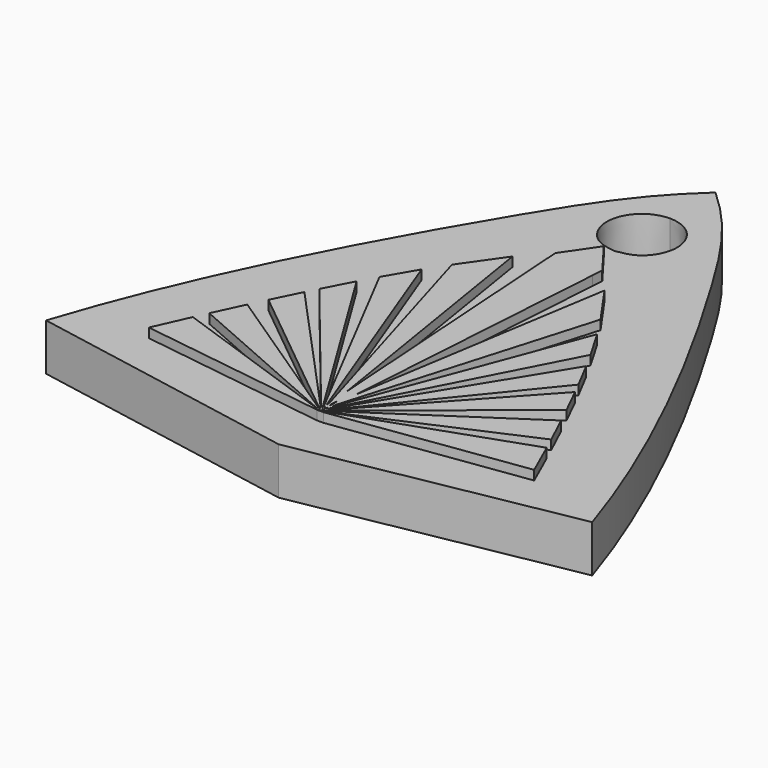
from build123d import *

# Parameters (mm, degrees)
F1_DEPTH = 5
F2_DEPTH = 6


# Not quite as in the source:
# - ends of sketch curves that miss each other by under 0.0002 mm in the source are joined
# - the dataset's text gives a spline's control points without its knots; the knots are read off the source's solid


with BuildPart() as f1:
    # F0 (on Top) → F1 (new body)
    with BuildSketch(Plane.XY):
        with BuildLine():
            add(Edge.make_bspline(
                [(0, 28.767477721), (-4.3973337825, 24.7953766473), (-10.7954077038, 15.1380571302), (-24.0578016888, -8.5453422723), (-29.069265, -23.969107)],
                knots=[0, 0, 0, 0, 0.3845016871, 1, 1, 1, 1], degree=3))
            Line((-29.069265, -23.969107), (-0.0365, -29.314396))
            Line((-0.0365, -29.314396), (29.069265, -23.969107))
            add(Edge.make_bspline(
                [(0, 28.767477721), (4.3973337825, 24.7953766473), (10.7954077038, 15.1380571302), (24.0578016888, -8.5453422723), (29.069265, -23.969107)],
                knots=[0, 0, 0, 0, 0.3845016871, 1, 1, 1, 1], degree=3))
        make_face()
        with BuildLine():
            Line((0.319138, -23.880866), (0.319138, -23.884253))
            Line((0.319138, -23.884253), (18.947309, -17.376961))
            add(Edge.make_bspline(
                [(20.618817, -21.132774), (20.455632, -20.760303), (20.108363, -19.967658), (19.551311, -18.715647), (19.15498, -17.837234), (18.947309, -17.376961)],
                knots=[0, 0, 0, 0, 1.219947, 2.596139, 4.110998, 4.110998, 4.110998, 4.110998], degree=3))
            Line((20.618817, -21.132774), (0.447831, -23.968919))
            Line((0.447831, -23.968919), (0.312364, -23.968919))
            Line((0.312364, -23.968919), (0.280003, -23.968919))
            Line((0.280003, -23.968919), (0.275111, -23.968919))
            Line((0.275111, -23.968919), (0.254791, -23.968919))
            Line((0.254791, -23.968919), (0.244631, -23.968919))
            Line((0.244631, -23.968919), (-0.019905, -23.968919))
            Line((-0.019905, -23.968919), (-0.030065, -23.968919))
            Line((-0.030065, -23.968919), (-0.04888, -23.968919))
            Line((-0.04888, -23.968919), (-0.054148, -23.968919))
            Line((-0.054148, -23.968919), (-0.086134, -23.968919))
            Line((-0.086134, -23.968919), (-0.2216, -23.968919))
            Line((-0.2216, -23.968919), (-20.392586, -21.132774))
            add(Edge.make_bspline(
                [(-18.721078, -17.376961), (-18.928749, -17.837234), (-19.32508, -18.715647), (-19.882132, -19.967658), (-20.229401, -20.760303), (-20.392586, -21.132774)],
                knots=[0, 0, 0, 0, 1.514859, 2.891051, 4.110998, 4.110998, 4.110998, 4.110998], degree=3))
            Line((-18.721078, -17.376961), (-0.092907, -23.884253))
            Line((-0.092907, -23.884253), (-0.092907, -23.880866))
            Line((-0.092907, -23.880866), (-18.083632, -15.981654))
            add(Edge.make_bspline(
                [(-16.595004, -12.792543), (-16.767405, -13.156812), (-17.107374, -13.875134), (-17.603121, -14.938403), (-17.925311, -15.637919), (-18.083632, -15.981654)],
                knots=[0, 0, 0, 0, 1.209017, 2.384129, 3.51946, 3.51946, 3.51946, 3.51946], degree=3))
            Line((-16.595004, -12.792543), (-0.09968, -23.772493))
            Line((-0.09968, -23.772493), (-0.101185, -23.736744))
            Line((-0.101185, -23.736744), (-15.752101, -11.0311))
            add(Edge.make_bspline(
                [(-14.292447, -8.070777), (-14.458037, -8.401363), (-14.788026, -9.060156), (-15.273718, -10.047373), (-15.593176, -10.704294), (-15.752101, -11.0311)],
                knots=[0, 0, 0, 0, 1.109215, 2.210448, 3.300648, 3.300648, 3.300648, 3.300648], degree=3))
            Line((-14.292447, -8.070777), (-0.111722, -23.597891))
            Line((-0.111722, -23.597891), (-0.113227, -23.56553))
            Line((-0.113227, -23.56553), (-13.678708, -6.854964))
            add(Edge.make_bspline(
                [(-12.106918, -3.854377), (-12.283656, -4.184869), (-12.638061, -4.847592), (-13.161704, -5.84798), (-13.506245, -6.519052), (-13.678708, -6.854964)],
                knots=[0, 0, 0, 0, 1.124341, 2.254598, 3.387391, 3.387391, 3.387391, 3.387391], degree=3))
            Line((-12.106918, -3.854377), (-0.126774, -23.361953))
            Line((-0.126774, -23.361953), (-0.136934, -23.211058))
            Line((-0.136934, -23.211058), (-11.115001, -2.041758))
            add(Edge.make_bspline(
                [(-9.227876, 1.200034), (-9.438006, 0.852886), (-9.864261, 0.148687), (-10.492017, -0.932835), (-10.905719, -1.669232), (-11.115001, -2.041758)],
                knots=[0, 0, 0, 0, 1.217356, 2.469433, 3.75129, 3.75129, 3.75129, 3.75129], degree=3))
            Line((-9.227876, 1.200034), (-0.164027, -22.805787))
            Line((-0.164027, -22.805787), (-0.194507, -22.35649))
            Line((-0.194507, -22.35649), (-7.79381, 3.443136))
            add(Edge.make_bspline(
                [(-4.787579, 7.734419), (-5.135061, 7.252834), (-5.826681, 6.294297), (-6.832139, 4.866004), (-7.477648, 3.910923), (-7.79381, 3.443136)],
                knots=[0, 0, 0, 0, 1.781576, 3.546009, 5.239803, 5.239803, 5.239803, 5.239803], degree=3))
            Line((-4.787579, 7.734419), (-0.367603, -19.764184))
            Line((-0.367603, -19.764184), (-2.305529, 9.216274))
            Line((-2.305529, 9.216274), (-2.378154, 10.418917))
            Line((-2.378154, 10.418917), (-2.359716, 10.440366))
            Line((-2.359716, 10.440366), (-2.381541, 10.440366))
            Line((-2.381541, 10.440366), (-0.010122, 13.91772))
            Line((-0.010122, 13.91772), (2.610782, 10.440366))
            Line((2.610782, 10.440366), (2.585946, 10.440366))
            Line((2.585946, 10.440366), (2.604761, 10.418917))
            Line((2.604761, 10.418917), (2.53176, 9.216274))
            Line((2.53176, 9.216274), (0.593834, -19.764184))
            Line((0.593834, -19.764184), (5.011929, 7.734419))
            add(Edge.make_bspline(
                [(8.020041, 3.443136), (7.703893, 3.910928), (7.058366, 4.866089), (6.052566, 6.294592), (5.359965, 7.252875), (5.011929, 7.734419)],
                knots=[0, 0, 0, 0, 1.693786, 3.458451, 5.240898, 5.240898, 5.240898, 5.240898], degree=3))
            Line((8.020041, 3.443136), (0.420738, -22.35649))
            Line((0.420738, -22.35649), (0.390258, -22.805787))
            Line((0.390258, -22.805787), (9.454106, 1.200034))
            add(Edge.make_bspline(
                [(11.341608, -2.041758), (11.132228, -1.669238), (10.718345, -0.932874), (10.090504, 0.148671), (9.664238, 0.852884), (9.454106, 1.200034)],
                knots=[0, 0, 0, 0, 1.281987, 2.534113, 3.751476, 3.751476, 3.751476, 3.751476], degree=3))
            Line((11.341608, -2.041758), (0.363164, -23.211058))
            Line((0.363164, -23.211058), (0.353004, -23.361953))
            Line((0.353004, -23.361953), (12.333149, -3.854377))
            add(Edge.make_bspline(
                [(13.904939, -6.854964), (13.732109, -6.519097), (13.386923, -5.848287), (12.86394, -4.84756), (12.509769, -4.184858), (12.333149, -3.854377)],
                knots=[0, 0, 0, 0, 1.133177, 2.263239, 3.387384, 3.387384, 3.387384, 3.387384], degree=3))
            Line((13.904939, -6.854964), (0.339458, -23.56553))
            Line((0.339458, -23.56553), (0.337576, -23.597891))
            Line((0.337576, -23.597891), (14.518678, -8.070777))
            add(Edge.make_bspline(
                [(15.978331, -11.0311), (15.819406, -10.704294), (15.499948, -10.047374), (15.014257, -9.060156), (14.684268, -8.401363), (14.518678, -8.070777)],
                knots=[0, 0, 0, 0, 1.0902, 2.191433, 3.300648, 3.300648, 3.300648, 3.300648], degree=3))
            Line((15.978331, -11.0311), (0.327792, -23.736744))
            Line((0.327792, -23.736744), (0.325911, -23.772493))
            Line((0.325911, -23.772493), (16.821235, -12.792543))
            add(Edge.make_bspline(
                [(18.309863, -15.981654), (18.151542, -15.637919), (17.829352, -14.938403), (17.333605, -13.875134), (16.993636, -13.156812), (16.821235, -12.792543)],
                knots=[0, 0, 0, 0, 1.135331, 2.310443, 3.51946, 3.51946, 3.51946, 3.51946], degree=3))
            Line((18.309863, -15.981654), (0.319138, -23.880866))
        make_face(mode=Mode.SUBTRACT)
        with BuildLine():
            add(Edge.make_bspline(
                [(-0.036575, 15.295228), (0.621493, 15.39784), (1.918116, 15.600022), (3.345493, 17.086348), (3.874317, 19.025119), (3.345531, 20.984289), (1.918153, 22.410914), (0.6214109026, 22.762095581), (-0.0367424704, 22.7620752759), (-0.0368262533, 22.7620752704)],
                knots=[0, 0, 0, 0, 1.951831, 3.845791, 5.797691, 7.749847, 9.643876, 11.595711, 11.5959595, 11.5959595, 11.5959595, 11.5959595], degree=3))
            add(Edge.make_bspline(
                [(-0.0368262533, 22.7620752704), (-0.6948437512, 22.7620322819), (-1.9914531815, 22.4108298617), (-3.418944, 20.984346), (-3.947897, 19.025119), (-3.418906, 17.086291), (-1.991357, 15.60004), (-0.694669, 15.397845), (-0.036575, 15.295228)],
                knots=[11.5959595, 11.5959595, 11.5959595, 11.5959595, 13.54764, 15.441797, 17.393979, 19.345905, 21.239993, 23.191919, 23.191919, 23.191919, 23.191919], degree=3))
        make_face(mode=Mode.SUBTRACT)
    extrude(amount=F1_DEPTH)

    # F0 (on Top) → F2 (join)
    with BuildSketch(Plane.XY):
        with BuildLine():
            Line((18.947309, -17.376961), (0.319138, -23.884253))
            Line((0.319138, -23.884253), (0.319138, -23.880866))
            Line((0.319138, -23.880866), (18.309863, -15.981654))
            add(Edge.make_bspline(
                [(18.309863, -15.981654), (18.151542, -15.637919), (17.829352, -14.938403), (17.333605, -13.875134), (16.993636, -13.156812), (16.821235, -12.792543)],
                knots=[0, 0, 0, 0, 1.135331, 2.310443, 3.51946, 3.51946, 3.51946, 3.51946], degree=3))
            Line((16.821235, -12.792543), (0.325911, -23.772493))
            Line((0.325911, -23.772493), (0.327792, -23.736744))
            Line((0.327792, -23.736744), (15.978331, -11.0311))
            add(Edge.make_bspline(
                [(15.978331, -11.0311), (15.819406, -10.704294), (15.499948, -10.047374), (15.014257, -9.060156), (14.684268, -8.401363), (14.518678, -8.070777)],
                knots=[0, 0, 0, 0, 1.0902, 2.191433, 3.300648, 3.300648, 3.300648, 3.300648], degree=3))
            Line((14.518678, -8.070777), (0.337576, -23.597891))
            Line((0.337576, -23.597891), (0.339458, -23.56553))
            Line((0.339458, -23.56553), (13.904939, -6.854964))
            add(Edge.make_bspline(
                [(13.904939, -6.854964), (13.732109, -6.519097), (13.386923, -5.848287), (12.86394, -4.84756), (12.509769, -4.184858), (12.333149, -3.854377)],
                knots=[0, 0, 0, 0, 1.133177, 2.263239, 3.387384, 3.387384, 3.387384, 3.387384], degree=3))
            Line((12.333149, -3.854377), (0.353004, -23.361953))
            Line((0.353004, -23.361953), (0.363164, -23.211058))
            Line((0.363164, -23.211058), (11.341608, -2.041758))
            add(Edge.make_bspline(
                [(11.341608, -2.041758), (11.132228, -1.669238), (10.718345, -0.932874), (10.090504, 0.148671), (9.664238, 0.852884), (9.454106, 1.200034)],
                knots=[0, 0, 0, 0, 1.281987, 2.534113, 3.751476, 3.751476, 3.751476, 3.751476], degree=3))
            Line((9.454106, 1.200034), (0.390258, -22.805787))
            Line((0.390258, -22.805787), (0.420738, -22.35649))
            Line((0.420738, -22.35649), (8.020041, 3.443136))
            add(Edge.make_bspline(
                [(8.020041, 3.443136), (7.703893, 3.910928), (7.058366, 4.866089), (6.052566, 6.294592), (5.359965, 7.252875), (5.011929, 7.734419)],
                knots=[0, 0, 0, 0, 1.693786, 3.458451, 5.240898, 5.240898, 5.240898, 5.240898], degree=3))
            Line((5.011929, 7.734419), (0.593834, -19.764184))
            Line((0.593834, -19.764184), (2.53176, 9.216274))
            Line((2.53176, 9.216274), (2.604761, 10.418917))
            Line((2.604761, 10.418917), (2.585946, 10.440366))
            Line((2.585946, 10.440366), (2.610782, 10.440366))
            Line((2.610782, 10.440366), (-0.010122, 13.91772))
            Line((-0.010122, 13.91772), (-2.381541, 10.440366))
            Line((-2.381541, 10.440366), (-2.359716, 10.440366))
            Line((-2.359716, 10.440366), (-2.378154, 10.418917))
            Line((-2.378154, 10.418917), (-2.305529, 9.216274))
            Line((-2.305529, 9.216274), (-0.367603, -19.764184))
            Line((-0.367603, -19.764184), (-4.787579, 7.734419))
            add(Edge.make_bspline(
                [(-4.787579, 7.734419), (-5.135061, 7.252834), (-5.826681, 6.294297), (-6.832139, 4.866004), (-7.477648, 3.910923), (-7.79381, 3.443136)],
                knots=[0, 0, 0, 0, 1.781576, 3.546009, 5.239803, 5.239803, 5.239803, 5.239803], degree=3))
            Line((-7.79381, 3.443136), (-0.194507, -22.35649))
            Line((-0.194507, -22.35649), (-0.164027, -22.805787))
            Line((-0.164027, -22.805787), (-9.227876, 1.200034))
            add(Edge.make_bspline(
                [(-9.227876, 1.200034), (-9.438006, 0.852886), (-9.864261, 0.148687), (-10.492017, -0.932835), (-10.905719, -1.669232), (-11.115001, -2.041758)],
                knots=[0, 0, 0, 0, 1.217356, 2.469433, 3.75129, 3.75129, 3.75129, 3.75129], degree=3))
            Line((-11.115001, -2.041758), (-0.136934, -23.211058))
            Line((-0.136934, -23.211058), (-0.126774, -23.361953))
            Line((-0.126774, -23.361953), (-12.106918, -3.854377))
            add(Edge.make_bspline(
                [(-12.106918, -3.854377), (-12.283656, -4.184869), (-12.638061, -4.847592), (-13.161704, -5.84798), (-13.506245, -6.519052), (-13.678708, -6.854964)],
                knots=[0, 0, 0, 0, 1.124341, 2.254598, 3.387391, 3.387391, 3.387391, 3.387391], degree=3))
            Line((-13.678708, -6.854964), (-0.113227, -23.56553))
            Line((-0.113227, -23.56553), (-0.111722, -23.597891))
            Line((-0.111722, -23.597891), (-14.292447, -8.070777))
            add(Edge.make_bspline(
                [(-14.292447, -8.070777), (-14.458037, -8.401363), (-14.788026, -9.060156), (-15.273718, -10.047373), (-15.593176, -10.704294), (-15.752101, -11.0311)],
                knots=[0, 0, 0, 0, 1.109215, 2.210448, 3.300648, 3.300648, 3.300648, 3.300648], degree=3))
            Line((-15.752101, -11.0311), (-0.101185, -23.736744))
            Line((-0.101185, -23.736744), (-0.09968, -23.772493))
            Line((-0.09968, -23.772493), (-16.595004, -12.792543))
            add(Edge.make_bspline(
                [(-16.595004, -12.792543), (-16.767405, -13.156812), (-17.107374, -13.875134), (-17.603121, -14.938403), (-17.925311, -15.637919), (-18.083632, -15.981654)],
                knots=[0, 0, 0, 0, 1.209017, 2.384129, 3.51946, 3.51946, 3.51946, 3.51946], degree=3))
            Line((-18.083632, -15.981654), (-0.092907, -23.880866))
            Line((-0.092907, -23.880866), (-0.092907, -23.884253))
            Line((-0.092907, -23.884253), (-18.721078, -17.376961))
            add(Edge.make_bspline(
                [(-18.721078, -17.376961), (-18.928749, -17.837234), (-19.32508, -18.715647), (-19.882132, -19.967658), (-20.229401, -20.760303), (-20.392586, -21.132774)],
                knots=[0, 0, 0, 0, 1.514859, 2.891051, 4.110998, 4.110998, 4.110998, 4.110998], degree=3))
            Line((-20.392586, -21.132774), (-0.2216, -23.968919))
            Line((-0.2216, -23.968919), (-0.086134, -23.968919))
            Line((-0.086134, -23.968919), (-0.054148, -23.968919))
            Line((-0.054148, -23.968919), (-0.04888, -23.968919))
            Line((-0.04888, -23.968919), (-0.030065, -23.968919))
            Line((-0.030065, -23.968919), (-0.019905, -23.968919))
            Line((-0.019905, -23.968919), (0.244631, -23.968919))
            Line((0.244631, -23.968919), (0.254791, -23.968919))
            Line((0.254791, -23.968919), (0.275111, -23.968919))
            Line((0.275111, -23.968919), (0.280003, -23.968919))
            Line((0.280003, -23.968919), (0.312364, -23.968919))
            Line((0.312364, -23.968919), (0.447831, -23.968919))
            Line((0.447831, -23.968919), (20.618817, -21.132774))
            add(Edge.make_bspline(
                [(20.618817, -21.132774), (20.455632, -20.760303), (20.108363, -19.967658), (19.551311, -18.715647), (19.15498, -17.837234), (18.947309, -17.376961)],
                knots=[0, 0, 0, 0, 1.219947, 2.596139, 4.110998, 4.110998, 4.110998, 4.110998], degree=3))
        make_face()
        Polygon((0.000415, -23.840226), (-0.013132, -23.830066), (-0.00824, -23.813133), (0.005306, -23.824798), align=None, mode=Mode.SUBTRACT)
        Polygon((-0.015014, -23.546715), (-0.023292, -23.531663), (-0.016519, -23.445115), (-0.002972, -23.472208), align=None, mode=Mode.SUBTRACT)
        Polygon((0.112175, -23.914733), (0.110669, -23.913227), (0.112175, -23.911346), (0.115561, -23.913227), align=None, mode=Mode.SUBTRACT)
        Polygon((0.042936, -23.867319), (0.027508, -23.859041), (0.034281, -23.846999), (0.047828, -23.859041), align=None, mode=Mode.SUBTRACT)
        Polygon((0.080189, -23.806359), (0.06288, -23.789426), (0.064761, -23.786039), (0.081695, -23.804478), align=None, mode=Mode.SUBTRACT)
        Polygon((0.183671, -23.867319), (0.178403, -23.859041), (0.191949, -23.846999), (0.198723, -23.859041), align=None, mode=Mode.SUBTRACT)
        Polygon((0.146041, -23.806359), (0.144536, -23.804478), (0.159588, -23.786039), (0.161469, -23.789426), align=None, mode=Mode.SUBTRACT)
        Polygon((0.032776, -23.753678), (0.013961, -23.735239), (0.017348, -23.724703), (0.034281, -23.746904), align=None, mode=Mode.SUBTRACT)
        Polygon((0.112175, -23.753678), (0.097123, -23.726584), (0.112175, -23.694223), (0.129108, -23.726584), align=None, mode=Mode.SUBTRACT)
        Polygon((0.208883, -23.724703), (0.212269, -23.735239), (0.193455, -23.753678), (0.190444, -23.746904), align=None, mode=Mode.SUBTRACT)
        Polygon((0.225816, -23.840226), (0.220548, -23.824798), (0.234471, -23.813133), (0.239363, -23.830066), align=None, mode=Mode.SUBTRACT)
        Polygon((0.080189, -23.629876), (0.06288, -23.672774), (0.042936, -23.638531), (0.057988, -23.587731), align=None, mode=Mode.SUBTRACT)
        Polygon((0.183671, -23.638531), (0.162975, -23.672774), (0.146041, -23.629876), (0.168243, -23.587731), align=None, mode=Mode.SUBTRACT)
        Polygon((0.112175, -23.541823), (0.090349, -23.478981), (0.112175, -23.399207), (0.135881, -23.478981), align=None, mode=Mode.SUBTRACT)
        Polygon((0.249523, -23.531663), (0.239363, -23.546715), (0.227698, -23.472208), (0.242749, -23.445115), align=None, mode=Mode.SUBTRACT)
        Polygon((0.046323, -23.1723), (0.024121, -23.306261), (0.000415, -23.240033), (0.013961, -23.062045), align=None, mode=Mode.SUBTRACT)
        Polygon((0.225816, -23.240033), (0.202109, -23.306261), (0.179908, -23.1723), (0.212269, -23.062045), align=None, mode=Mode.SUBTRACT)
        Polygon((0.162975, -22.438146), (0.112175, -22.754987), (0.061375, -22.438146), (0.112175, -21.786777), align=None, mode=Mode.SUBTRACT)
    extrude(amount=F2_DEPTH)


solid = f1.part
